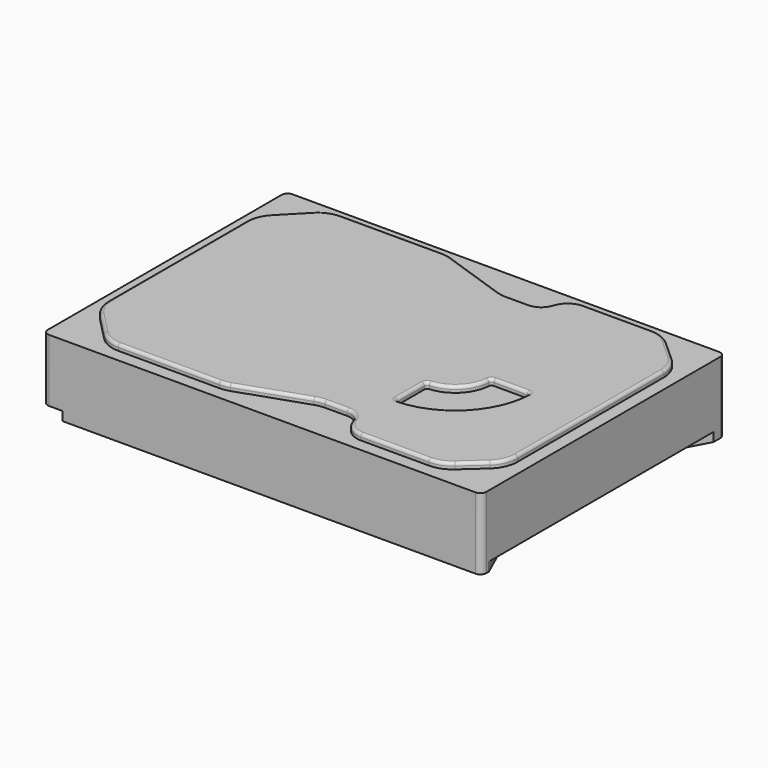
from build123d import *

# Parameters (mm, degrees)
F0_W      = 147
F0_H      = 102
F1_DEPTH  = 26
F2_R      = 2
F3_R      = 25.1169689263
F4_DEPTH  = 3
F6_DEPTH  = 2
F7_R      = 25.1169689263
F7_W      = 7.9772167655
F7_H      = 4.1224605193
F7_W_2    = 4.1224605193
F7_H_2    = 7.9772167655
F8_DEPTH  = 2
F9_SIZE2  = 1.99999
F9_SIZE   = 6.99999
F10_R     = 5
F12_DEPTH = 2
F13_R     = 1


# Not quite as in the source:
# - a fillet or chamfer is up to 0.001 mm smaller than in the source, because OpenCascade refuses the exact size


with BuildPart() as f1:
    # F0 (on Top) → F1 (new body)
    with BuildSketch(Plane.XY):
        with Locations((73.5, 51)):
            Rectangle(F0_W, F0_H)
    extrude(amount=F1_DEPTH)

    # F2
    f2_edges = [f1.edges().sort_by_distance(p)[0] for p in [
        (0, 0, 13),
        (147, 0, 13),
        (147, 102, 13),
        (0, 102, 13),
    ]]
    fillet(f2_edges, radius=F2_R)

    # F3 (on face) → F4 (cut)
    with BuildSketch(Plane(origin=(0, 0, 0), x_dir=(1, 0, 0), z_dir=(0, 0, -1))):
        with BuildLine():
            Line((144, -3), (6.5606157295, -3))
            Line((6.5606157295, -3), (6.5606157295, 0))
            Line((6.5606157295, 0), (2, 0))
            ThreePointArc((2, 0), (0.5857864376, -0.5857864376), (0, -2))
            Line((0, -2), (0, -100))
            ThreePointArc((0, -100), (0.5857864376, -101.4142135624), (2, -102))
            Line((2, -102), (14.2296897247, -102))
            Line((14.2296897247, -102), (14.2296897247, -99))
            Line((14.2296897247, -99), (145, -99))
            Line((145, -99), (137.9531513453, -85.8632188108))
            Line((137.9531513453, -85.8632188108), (137.9531513453, -16.6260308719))
            Line((137.9531513453, -16.6260308719), (144, -3))
        make_face()
        with Locations((98.0989858508, -50.0876903534)):
            Circle(F3_R, mode=Mode.SUBTRACT)
        Polygon((147, -97.1357934826), (147, -3), (140.9531513453, -16.6260308719), (140.9531513453, -85.8632188108), align=None)
    extrude(amount=-F4_DEPTH, mode=Mode.SUBTRACT)

    # F5 (on face) → F6 (join)
    with BuildSketch(Plane(origin=(0, 0, 3), x_dir=(1, 0, 0), z_dir=(0, 0, -1))):
        with BuildLine():
            Line((14.2296897247, -99), (55.0723448396, -99))
            Line((55.0723448396, -99), (55.0723448396, -42.5031647924))
            Line((55.0723448396, -42.5031647924), (23.9577665925, -28.1695667654))
            Line((23.9577665925, -28.1695667654), (0, -28.1695667654))
            Line((0, -28.1695667654), (0, -100))
            ThreePointArc((0, -100), (0.5857864376, -101.4142135624), (2, -102))
            Line((2, -102), (14.2296897247, -102))
            Line((14.2296897247, -102), (14.2296897247, -99))
        make_face()
    extrude(amount=F6_DEPTH)

    # F7 (on face) → F8 (join)
    with BuildSketch(Plane(origin=(0, 0, 3), x_dir=(1, 0, 0), z_dir=(0, 0, -1))):
        Polygon((68.5814172029, -11.8443537503), (68.5814172029, -22.7281169246), (68.5814172029, -36.7360695054), (68.5814172029, -79.8824131489), (92.3246070743, -79.8824131489), (108.6435541511, -79.8824131489), (128.9916932583, -79.8824131489), (128.9916932583, -11.8443537503), align=None)
        with Locations((98.0989858508, -50.0876903534)):
            Circle(F7_R, mode=Mode.SUBTRACT)
        Polygon((68.5814172029, -36.7360695054), (68.5814172029, -22.7281169246), (61.3132603467, -22.7281169246), (61.3132603467, -26.8505774438), (61.3132603467, -32.6136089861), (61.3132603467, -36.7360695054), align=None)
        Polygon((108.6435541511, -79.8824131489), (92.3246070743, -79.8824131489), (92.3246070743, -85.6698147568), (96.4470675935, -85.6698147568), (104.5210936318, -85.6698147568), (108.6435541511, -85.6698147568), align=None)
        with Locations((57.3246519639, -24.7893471842)):
            Rectangle(F7_W, F7_H)
        with Locations((57.3246519639, -34.6748392458)):
            Rectangle(F7_W, F7_H)
        with Locations((94.3858373339, -89.6584231396)):
            Rectangle(F7_W_2, F7_H_2)
        with Locations((106.5823238914, -89.6584231396)):
            Rectangle(F7_W_2, F7_H_2)
    extrude(amount=F8_DEPTH)

    # F9 (size 7 and 2 in the source; OpenCascade refuses exactly that, so slightly less here)
    f9_edges = [f1.edges().sort_by_distance(p)[0] for p in [
        (53.336044, 24.789347, 1),
        (53.336044, 34.674839, 1),
        (94.385837, 93.647032, 1),
        (106.582324, 93.647032, 1),
    ]]
    f9_side = f1.faces().sort_by_distance((69.695664, 17.286235, 1))[0]
    chamfer(f9_edges, length=F9_SIZE, length2=F9_SIZE2, reference=f9_side)

    # F10
    f10_edges = [f1.edges().sort_by_distance(p)[0] for p in [
        (68.581417, 11.844354, 2),
        (128.991693, 11.844354, 2),
        (128.991693, 79.882413, 2),
        (68.581417, 79.882413, 2),
    ]]
    fillet(f10_edges, radius=F10_R)

    # F11 (on face) → F12 (cut)
    with BuildSketch(Plane.XY.offset(26)):
        with BuildLine():
            ThreePointArc((2, 102), (0.5857864376, 101.4142135624), (0, 100))
            Line((0, 100), (0, 2))
            ThreePointArc((0, 2), (0.5857864376, 0.5857864376), (2, 0))
            Line((2, 0), (145, 0))
            ThreePointArc((145, 0), (146.4142135624, 0.5857864376), (147, 2))
            Line((147, 2), (147, 100))
            ThreePointArc((147, 100), (146.4142135624, 101.4142135624), (145, 102))
            Line((145, 102), (2, 102))
        make_face()
        with BuildLine():
            Line((4.2258142494, 22.0722364937), (4.2258142494, 51))
            Line((4.2258142494, 51), (4.2258142494, 79.9277635063))
            ThreePointArc((4.2258142494, 79.9277635063), (4.9610816932, 83.691369578), (7.058760382, 86.9015242465))
            Line((7.058760382, 86.9015242465), (14.6935671534, 94.7479464908))
            ThreePointArc((14.6935671534, 94.7479464908), (17.9707371795, 96.986612342), (21.8606210208, 97.7741857506))
            Line((21.8606210208, 97.7741857506), (55.7528358207, 97.7741857506))
            ThreePointArc((55.7528358207, 97.7741857506), (57.3980089851, 97.6379277008), (58.9983485321, 97.2328668025))
            Line((58.9983485321, 97.2328668025), (80.9614386994, 89.6967750441))
            ThreePointArc((80.9614386994, 89.6967750441), (82.5617782464, 89.2917141458), (84.2069514108, 89.1554560959))
            Line((84.2069514108, 89.1554560959), (91.6838514243, 89.1554560959))
            ThreePointArc((91.6838514243, 89.1554560959), (94.5898246688, 90.0866332315), (96.4134075766, 92.533328295))
            Line((96.4134075766, 92.533328295), (96.5889555539, 93.0451646719))
            ThreePointArc((96.5889555539, 93.0451646719), (99.1419716248, 96.4705377609), (103.2103341671, 97.7741857506))
            Line((103.2103341671, 97.7741857506), (125.9630903806, 97.7741857506))
            ThreePointArc((125.9630903806, 97.7741857506), (129.5503496104, 97.1086150968), (132.660093946, 95.2004999942))
            Line((132.660093946, 95.2004999942), (139.4711893161, 89.0582969469))
            ThreePointArc((139.4711893161, 89.0582969469), (141.9111993671, 85.6958456652), (142.7741857506, 81.6319827033))
            Line((142.7741857506, 81.6319827033), (142.7741857506, 51))
            Line((142.7741857506, 51), (142.7741857506, 20.3680172967))
            ThreePointArc((142.7741857506, 20.3680172967), (141.9111993671, 16.3041543348), (139.4711893161, 12.9417030531))
            Line((139.4711893161, 12.9417030531), (132.660093946, 6.7995000058))
            ThreePointArc((132.660093946, 6.7995000058), (129.5503496104, 4.8913849032), (125.9630903806, 4.2258142494))
            Line((125.9630903806, 4.2258142494), (103.2103341671, 4.2258142494))
            ThreePointArc((103.2103341671, 4.2258142494), (99.1419716248, 5.5294622391), (96.5889555539, 8.9548353281))
            Line((96.5889555539, 8.9548353281), (96.4134075766, 9.466671705))
            ThreePointArc((96.4134075766, 9.466671705), (94.5898246688, 11.9133667685), (91.6838514243, 12.8445439041))
            Line((91.6838514243, 12.8445439041), (84.2069514108, 12.8445439041))
            ThreePointArc((84.2069514108, 12.8445439041), (82.5617782464, 12.7082858542), (80.9614386994, 12.3032249559))
            Line((80.9614386994, 12.3032249559), (58.9983485321, 4.7671331975))
            ThreePointArc((58.9983485321, 4.7671331975), (57.3980089851, 4.3620722992), (55.7528358207, 4.2258142494))
            Line((55.7528358207, 4.2258142494), (21.8606210208, 4.2258142494))
            ThreePointArc((21.8606210208, 4.2258142494), (17.9707371795, 5.013387658), (14.6935671534, 7.2520535092))
            Line((14.6935671534, 7.2520535092), (7.058760382, 15.0984757535))
            ThreePointArc((7.058760382, 15.0984757535), (4.9610816932, 18.308630422), (4.2258142494, 22.0722364937))
        make_face(mode=Mode.SUBTRACT)
        with BuildLine():
            ThreePointArc((99.0220627739, 38.1232459871), (98.3651864651, 37.8055751771), (98.0989858508, 37.1262089566))
            Line((98.0989858508, 37.1262089566), (98.0989858508, 25.9914626364))
            ThreePointArc((98.0989858508, 25.9914626364), (98.4066942145, 25.269844808), (99.1404504313, 24.9923226619))
            ThreePointArc((99.1404504313, 24.9923226619), (115.8593649014, 32.3273113028), (123.1943535423, 49.0462257729))
            ThreePointArc((123.1943535423, 49.0462257729), (122.9168313962, 49.7799819897), (122.1952135678, 50.0876903534))
            Line((122.1952135678, 50.0876903534), (111.0604672476, 50.0876903534))
            ThreePointArc((111.0604672476, 50.0876903534), (110.3811010271, 49.8214897391), (110.0634302171, 49.1646134303))
            ThreePointArc((110.0634302171, 49.1646134303), (106.584267225, 41.6024089792), (99.0220627739, 38.1232459871))
        make_face()
    extrude(amount=-F12_DEPTH, mode=Mode.SUBTRACT)

    # F13
    f13_edges = [f1.edges().sort_by_distance(p)[0] for p in [
        (141.911199, 85.695846, 26),
        (142.774186, 51, 26),
        (141.911199, 16.304154, 26),
        (136.065642, 9.870602, 26),
        (129.55035, 4.891385, 26),
        (114.586712, 4.225814, 26),
        (99.141972, 5.529462, 26),
        (96.501182, 9.210754, 26),
        (94.589825, 11.913367, 26),
        (87.945401, 12.844544, 26),
        (82.561778, 12.708286, 26),
        (69.979894, 8.535179, 26),
        (57.398009, 4.362072, 26),
        (38.806728, 4.225814, 26),
        (17.970737, 5.013388, 26),
        (10.876164, 11.175265, 26),
        (4.961082, 18.30863, 26),
        (4.225814, 51, 26),
        (4.961082, 83.69137, 26),
        (10.876164, 90.824735, 26),
        (17.970737, 96.986612, 26),
        (38.806728, 97.774186, 26),
        (57.398009, 97.637928, 26),
        (69.979894, 93.464821, 26),
        (82.561778, 89.291714, 26),
        (87.945401, 89.155456, 26),
        (94.589825, 90.086633, 26),
        (96.501182, 92.789246, 26),
        (99.141972, 96.470538, 26),
        (114.586712, 97.774186, 26),
        (129.55035, 97.108615, 26),
        (136.065642, 92.129398, 26),
        (106.584267, 41.602409, 26),
        (98.365186, 37.805575, 26),
        (98.098986, 31.558836, 26),
        (98.406694, 25.269845, 26),
        (115.859365, 32.327311, 26),
        (122.916831, 49.779982, 26),
        (116.62784, 50.08769, 26),
        (110.381101, 49.82149, 26),
    ]]
    fillet(f13_edges, radius=F13_R)


solid = f1.part
